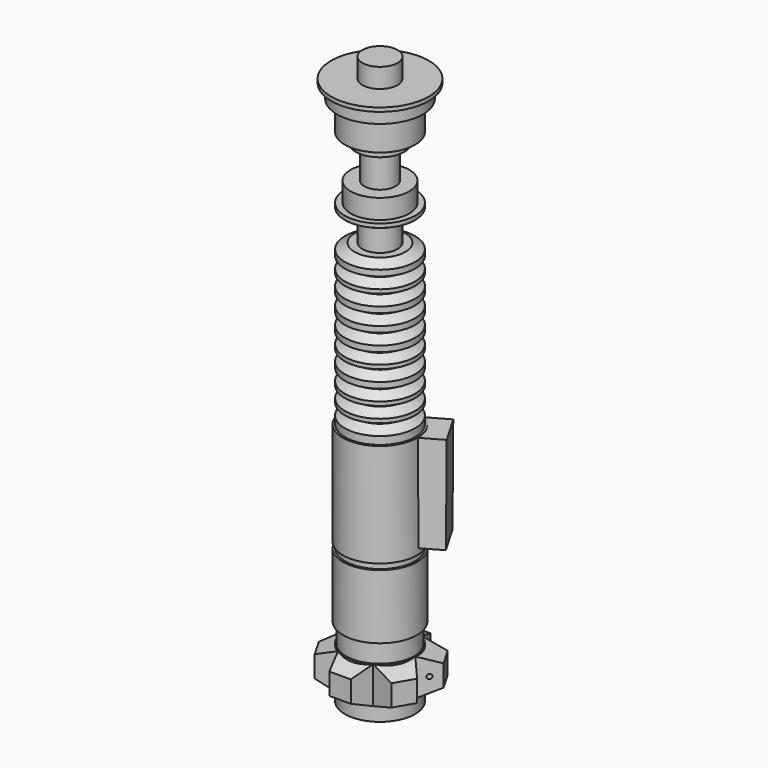
from build123d import *

# Parameters (mm, degrees)
F0_W      = 9
F0_H      = 10
F0_W_2    = 18
F0_H_2    = 4
F0_W_3    = 8
F0_H_3    = 17
F0_H_4    = 13
F0_H_5    = 3
F0_H_6    = 2
F0_H_7    = 1.8402965188
F2_W      = 18
F2_H      = 3
F2_W_2    = 17.5
F2_H_2    = 10
F10_W     = 18
F10_H     = 19
F15_W     = 18.0965775698
F15_H     = 19
F20_W     = 18
F20_H     = 19
F22_W     = 11
F22_H     = 11
F25_W     = 18
F25_H     = 19
F27_W     = 11
F27_H     = 11
F30_W     = 18
F30_H     = 19
F32_W     = 11
F32_H     = 11
F35_W     = 18
F35_H     = 19
F37_W     = 11
F37_H     = 11
F41_R     = 1.1953319017
F42_DEPTH = 43.6332552472
F4_W      = 18
F4_H      = 7
F47_DEPTH = 12


with BuildPart() as f1:
    # F0 (on Front) → F1 (revolve)
    with BuildSketch(Plane.XZ):
        with Locations((13.5, -5)):
            Rectangle(F0_W, F0_H)
        with Locations((18, -163.9402965188)):
            Rectangle(F0_W_2, F0_H_2)
        Polygon((34, -10), (18, -10), (9, -10), (9, -12), (31, -12), (34, -12), align=None)
        Polygon((31, -12), (9, -12), (9, -19), (27, -19), (31, -19), align=None)
        Polygon((27, -19), (9, -19), (9, -34), (21.5, -34), (27, -34), align=None)
        Polygon((21.5, -34), (9, -34), (9, -39), (17, -39), (21.5, -39), align=None)
        with Locations((13, -47.5)):
            Rectangle(F0_W_3, F0_H_3)
        Polygon((17, -56), (9, -56), (9, -66), (24, -66), (24, -56), align=None)
        Polygon((24, -66), (9, -66), (9, -68), (21.5, -68), (27, -68), (27, -66), align=None)
        Polygon((21.5, -68), (9, -68), (9, -71), (18, -71), (21.5, -71), align=None)
        with Locations((13.5, -77.5)):
            Rectangle(F0_W, F0_H_4)
        Polygon((18, -84), (9, -84), (9, -86.9), (27, -86.9), (21.9770526581, -84), align=None)
        with Locations((18, -88.4)):
            Rectangle(F0_W_2, F0_H_5)
        Polygon((27, -89.9), (9, -89.9), (9, -92.8), (21.9770526581, -92.8), align=None)
        Polygon((21.9770526581, -92.8), (9, -92.8), (9, -95.7), (27, -95.7), align=None)
        with Locations((18, -96.7)):
            Rectangle(F0_W_2, F0_H_6)
        Polygon((27, -97.7), (9, -97.7), (9, -100.6), (21.9770526581, -100.6), align=None)
        Polygon((21.9770526581, -100.6), (9, -100.6), (9, -103.5), (27, -103.5), align=None)
        with Locations((18, -105)):
            Rectangle(F0_W_2, F0_H_5)
        Polygon((27, -106.5), (9, -106.5), (9, -109.4), (21.9770526581, -109.4), align=None)
        Polygon((21.9770526581, -109.4), (9, -109.4), (9, -112.3), (27, -112.3), align=None)
        with Locations((18, -113.8)):
            Rectangle(F0_W_2, F0_H_5)
        Polygon((27, -115.3), (9, -115.3), (9, -118.2), (21.9770526581, -118.2), align=None)
        Polygon((21.9770526581, -118.2), (9, -118.2), (9, -121.1), (27, -121.1), align=None)
        with Locations((18, -122.6)):
            Rectangle(F0_W_2, F0_H_5)
        Polygon((27, -129.7402965188), (22.1153599298, -126.9201482594), (21.9770526581, -127), (27, -129.9), align=None)
        with Locations((18, -130.8201482594)):
            Rectangle(F0_W_2, F0_H_7)
        Polygon((27, -131.7402965188), (9, -131.7402965188), (9, -134.6402965188), (21.9770526581, -134.6402965188), align=None)
        Polygon((21.9770526581, -134.6402965188), (9, -134.6402965188), (9, -137.5402965188), (27, -137.5402965188), align=None)
        with Locations((18, -139.0402965188)):
            Rectangle(F0_W_2, F0_H_5)
        Polygon((27, -140.5402965188), (9, -140.5402965188), (9, -143.4402965188), (21.9770526581, -143.4402965188), align=None)
        Polygon((21.9770526581, -143.4402965188), (9, -143.4402965188), (9, -146.3402965188), (27, -146.3402965188), align=None)
        with Locations((18, -147.3402965188)):
            Rectangle(F0_W_2, F0_H_6)
        Polygon((27, -148.3402965188), (9, -148.3402965188), (9, -151.2402965188), (21.9770526581, -151.2402965188), align=None)
        Polygon((21.9770526581, -151.2402965188), (9, -151.2402965188), (9, -154.1402965188), (27, -154.1402965188), align=None)
        with Locations((18, -155.1402965188)):
            Rectangle(F0_W_2, F0_H_6)
        Polygon((27, -156.1402965188), (9, -156.1402965188), (9, -159.0402965188), (21.9770526581, -159.0402965188), align=None)
        Polygon((21.9770526581, -159.0402965188), (9, -159.0402965188), (9, -161.9402965188), (27, -161.9402965188), align=None)
        Polygon((27, -124.1), (9, -124.1), (9, -127), (21.9770526581, -127), (22.1153599298, -126.9201482594), align=None)
        Polygon((21.9770526581, -127), (9, -127), (9, -129.9), (27, -129.9), align=None)
    revolve(axis=Axis((9, 0, -82.9701482594), (0, 0, -1)))

    # F2 (on Front) → F3 (revolve)
    with BuildSketch(Plane.XZ):
        Polygon((27, -165.9402965188), (9, -165.9402965188), (9, -218.9402965188), (27, -218.9402965188), (28, -218.9402965188), (28, -165.9402965188), align=None)
        with Locations((18, -220.4402965188)):
            Rectangle(F2_W, F2_H)
        Polygon((27, -221.9402965188), (9, -221.9402965188), (9, -254.9402965188), (26.5, -254.9402965188), (28, -254.9402965188), (28, -221.9402965188), align=None)
        with Locations((17.75, -259.9402965188)):
            Rectangle(F2_W_2, F2_H_2)
    revolve(axis=Axis((9, 0, -192.4402965188), (0, 0, -1)))

    # F4 (on Front) → F5 (revolve)
    with BuildSketch(Plane.XZ):
        Polygon((26.5, -264.9402965188), (9, -264.9402965188), (9, -283.9402965188), (27, -283.9402965188), (27, -264.9402965188), align=None)
    revolve(axis=Axis((9, 0, -274.4402965188), (0, 0, -1)))

    # F10 (on 3pt) → F13 section 0
    with BuildSketch(Plane(origin=(20.25, 11.6913429511, 0), x_dir=(0.5, -0.8660254038, 0), z_dir=(-0.8660254038, -0.5, 0))):
        with Locations((4.5, -274.4402965188)):
            Rectangle(F10_W, F10_H)
    # F12 (on offset) → F13 section 1
    with BuildSketch(Plane(origin=(29.7762794416, 17.1913429511, 0), x_dir=(0.5, -0.8660254038, 0), z_dir=(-0.8660254038, -0.5, 0))):
        Polygon((10, -268.9402965188), (4.5, -268.9402965188), (-1, -268.9402965188), (-1, -279.9402965188), (10, -279.9402965188), align=None)
    loft()

    # F15 (on 3pt) → F18 section 0
    with BuildSketch(Plane(origin=(20.25, -11.6913429511, 0), x_dir=(-0.5, -0.8660254038, 0), z_dir=(-0.8660254038, 0.5, 0))):
        with Locations((-4.5482887849, -274.4402965188)):
            Rectangle(F15_W, F15_H)
    # F17 (on offset) → F18 section 1
    with BuildSketch(Plane(origin=(29.7762794416, -17.1913429511, 0), x_dir=(-0.5, -0.8660254038, 0), z_dir=(-0.8660254038, 0.5, 0))):
        Polygon((0.9517112151, -268.9402965188), (-4.5482887849, -268.9402965188), (-10.0482887849, -268.9402965188), (-10.0482887849, -279.9402965188), (0.9517112151, -279.9402965188), align=None)
    loft()

    # F20 (on 3pt) → F23 section 0
    with BuildSketch(Plane.XZ.offset(15.5884572681)):
        with Locations((9, -274.4402965188)):
            Rectangle(F20_W, F20_H)
    # F22 (on offset) → F23 section 1
    with BuildSketch(Plane.XZ.offset(25.5884572681)):
        with Locations((9, -274.4402965188)):
            Rectangle(F22_W, F22_H)
    loft()

    # F25 (on 3pt) → F28 section 0
    with BuildSketch(Plane(origin=(-6.75, -3.897114317, 0), x_dir=(-0.5, 0.8660254038, 0), z_dir=(0.8660254038, 0.5, 0))):
        with Locations((-4.5, -274.4402965188)):
            Rectangle(F25_W, F25_H)
    # F27 (on offset) → F28 section 1
    with BuildSketch(Plane(origin=(-15.4102540378, -8.897114317, 0), x_dir=(-0.5, 0.8660254038, 0), z_dir=(0.8660254038, 0.5, 0))):
        with Locations((-4.5, -274.4402965188)):
            Rectangle(F27_W, F27_H)
    loft()

    # F30 (on 3pt) → F33 section 0
    with BuildSketch(Plane(origin=(-6.75, 3.897114317, 0), x_dir=(0.5, 0.8660254038, 0), z_dir=(0.8660254038, -0.5, 0))):
        with Locations((4.5, -274.4402965188)):
            Rectangle(F30_W, F30_H)
    # F32 (on offset) → F33 section 1
    with BuildSketch(Plane(origin=(-15.4102540378, 8.897114317, 0), x_dir=(0.5, 0.8660254038, 0), z_dir=(0.8660254038, -0.5, 0))):
        with Locations((4.5, -274.4402965188)):
            Rectangle(F32_W, F32_H)
    loft()

    # F35 (on 3pt) → F38 section 0
    with BuildSketch(Plane(origin=(0, 15.5884572681, 0), x_dir=(-1, 0, 0), z_dir=(0, 1, 0))):
        with Locations((-9, -274.4402965188)):
            Rectangle(F35_W, F35_H)
    # F37 (on offset) → F38 section 1
    with BuildSketch(Plane(origin=(0, 25.5884572681, 0), x_dir=(-1, 0, 0), z_dir=(0, 1, 0))):
        with Locations((-9, -274.4402965188)):
            Rectangle(F37_W, F37_H)
    loft()

    # F41 (on 3pt) → F42 (cut, through all)
    with BuildSketch(Plane(origin=(6.7360005614, -11.6670952121, 0), x_dir=(0.8660254038, 0.5, 0), z_dir=(0.5, -0.8660254038, 0))):
        with Locations((28.9043522787, -274.4402965188)):
            Circle(F41_R)
    extrude(amount=-F42_DEPTH, mode=Mode.SUBTRACT)

    # F4 (on Front) → F43 (revolve)
    with BuildSketch(Plane.XZ):
        with Locations((18, -287.4402965188)):
            Rectangle(F4_W, F4_H)
    revolve(axis=Axis((9, 0, -287.4402965188), (0, 0, -1)))

    # F46 (on face) → F47 (join)
    with BuildSketch(Plane(origin=(21.8268516477, 12.7376953946, -0.178333724), x_dir=(0.5040000484, -0.8636938082, -0.0041178731), z_dir=(-0.8636649816, -0.5040168704, 0.0070564731))):
        Polygon((-3.7806784788, -215.8612271244), (5.2193215212, -215.8612271244), (14.2193215212, -215.8612271244), (14.2193215212, -165.9422449666), (-3.7806784788, -166.0163654656), align=None)
    extrude(amount=-F47_DEPTH)


solid = f1.part
